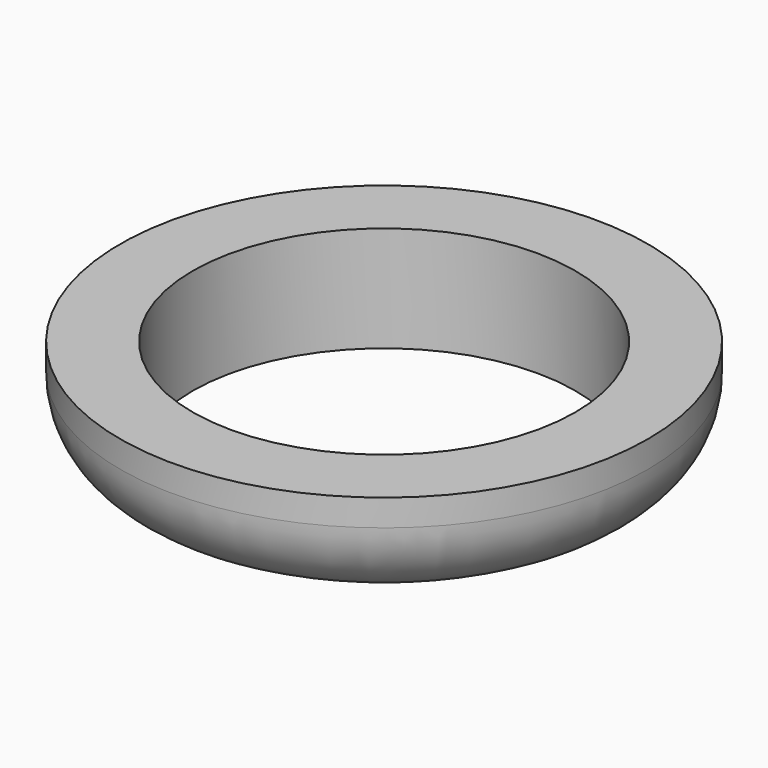
from build123d import *

# Parameters (mm, degrees)
F0_R     = 10
F0_R_2   = 7.25
F1_DEPTH = 4


# Not quite as in the source:
# - a fillet or chamfer that OpenCascade refuses, or shapes differently, is made with other operations: its cross-section is extruded or revolved along the edge and cut away or added


with BuildPart() as f1:
    # F0 (on Top) → F1 (new body)
    with BuildSketch(Plane.XY):
        Circle(F0_R)
        Circle(F0_R_2, mode=Mode.SUBTRACT)
    extrude(amount=-F1_DEPTH)

    # F2: fillet of radius 3 on 1 edges, made by hand

    # F2_s1 → F2_t2 (revolve, cut)
    with BuildSketch(Plane.XZ):
        with BuildLine():
            ThreePointArc((10, -1.0104348142), (9.2079402166, -3.0414444154), (7.25, -4))
            Line((7.25, -4), (10, -4))
            Line((10, -4), (10, -1.0104348142))
        make_face()
    revolve(axis=Axis((0, 0, -4), (0, 0, 1)), mode=Mode.SUBTRACT)


solid = f1.part
